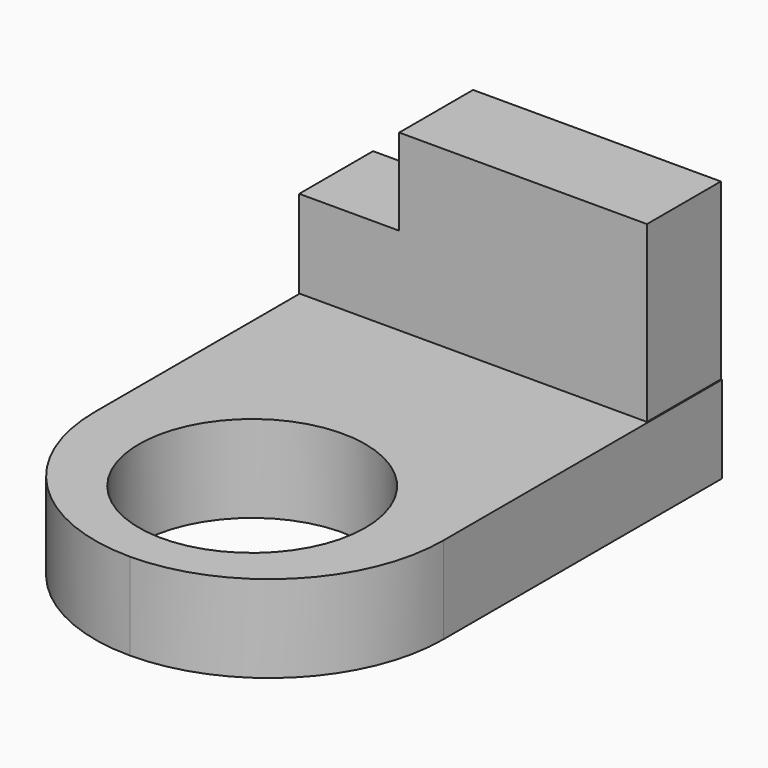
from build123d import *

# Parameters (mm, degrees)
F0_W     = 50.8
F0_H     = 76.2
F1_DEPTH = 12.7
F2_R     = 25.4
F3_R     = 25.39999
F4_W     = 50.7186688483
F4_H     = 13.4670715779
F5_DEPTH = 38.1
F6_W     = 14.5849827677
F6_H     = 12.6033662766
F7_DEPTH = 13.4680715779
F8_R     = 16.5120085349
F9_DEPTH = 38.101


# Not quite as in the source:
# - a fillet or chamfer is up to 0.001 mm smaller than in the source, because OpenCascade refuses the exact size


with BuildPart() as f1:
    # F0 (on Top) → F1 (new body)
    with BuildSketch(Plane.XY):
        Rectangle(F0_W, F0_H)
    extrude(amount=F1_DEPTH)

    # F2
    f2_edges = [f1.edges().sort_by_distance(p)[0] for p in [
        (25.4, -38.1, 6.35),
    ]]
    fillet(f2_edges, radius=F2_R)

    # F3 (radius 25.4 in the source; OpenCascade refuses exactly that, so slightly less here)
    f3_edges = [f1.edges().sort_by_distance(p)[0] for p in [
        (-25.4, -38.1, 6.35),
    ]]
    fillet(f3_edges, radius=F3_R)

    # F4 (on Top) → F5 (join)
    with BuildSketch(Plane.XY):
        with Locations((-0.1172143966, 31.366464211)):
            Rectangle(F4_W, F4_H)
    extrude(amount=F5_DEPTH)

    # F6 (on face) → F7 (cut, through all)
    with BuildSketch(Plane.XZ.offset(-24.6329284221)):
        with Locations((-18.1840574369, 31.7983168617)):
            Rectangle(F6_W, F6_H)
    extrude(amount=-F7_DEPTH, mode=Mode.SUBTRACT)

    # F8 (on Top) → F9 (cut, through all)
    with BuildSketch(Plane.XY):
        with Locations((0, -15.7830994576)):
            Circle(F8_R)
    extrude(amount=F9_DEPTH, mode=Mode.SUBTRACT)


solid = f1.part
